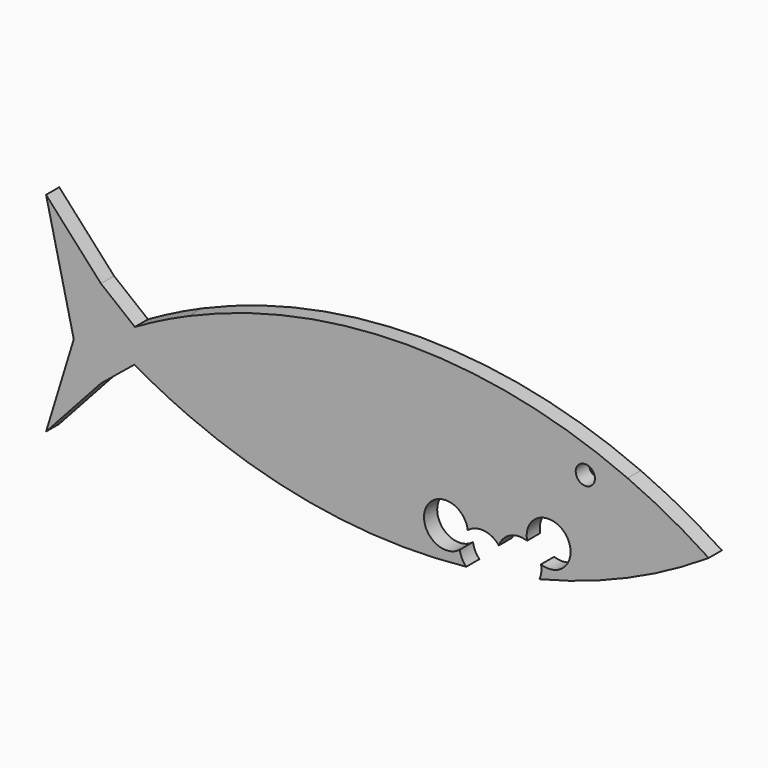
from build123d import *

# Parameters (mm, degrees)
F0_R     = 1.75
F1_DEPTH = 3


# Not quite as in the source:
# - a feature names something its author has since deleted; it is built from what else it names


with BuildPart() as f1:
    # F0 (on Front) → F1 (new body)
    with BuildSketch(Plane.XZ):
        with BuildLine():
            Line((0, 16), (0, 0))
            Line((0, 0), (43.6382221521, 0))
            ThreePointArc((43.6382221521, 0), (43.870370626, 0.294923121), (44.1291400161, 0.5667888304))
            ThreePointArc((44.1291400161, 0.5667888304), (41.7991534918, 8.3522131948), (44.5474305371, 16))
            Line((44.5474305371, 16), (0, 16))
        make_face()
        with BuildLine():
            ThreePointArc((-9.8901239272, 4.9856294086), (-5.0141391128, 2.3557845503), (0, 0))
            Line((0, 0), (0, 16))
            ThreePointArc((0, 16), (-4.9775998147, 13.6626256025), (-9.8191881817, 11.0551668638))
            ThreePointArc((-9.8191881817, 11.0551668638), (-12.3290859965, 9.5638999576), (-14.7943813031, 8))
            ThreePointArc((-14.7943813031, 8), (-12.3639476772, 6.4575177277), (-9.8901239272, 4.9856294086))
        make_face()
        with BuildLine():
            Line((43.6382221521, 0), (0, 0))
            ThreePointArc((0, 0), (24.7921839108, -7.1853331257), (50.5976363139, -7.7853510181))
            ThreePointArc((50.5976363139, -7.7853510181), (49.8103733831, -6.7032232406), (49.4240926583, -5.4219853039))
            ThreePointArc((49.4240926583, -5.4219853039), (44.1587611024, -5.2426073702), (43.6382221521, 0))
        make_face()
        with BuildLine():
            ThreePointArc((80, 16), (40, 24.3484861009), (0, 16))
            Line((0, 16), (44.5474305371, 16))
            ThreePointArc((44.5474305371, 16), (54.7943813031, 21), (65.041332069, 16))
            Line((65.041332069, 16), (80, 16))
        make_face()
        with BuildLine():
            Line((-16, -0.0001621457), (-9.8901239272, 4.9856294086))
            ThreePointArc((-9.8901239272, 4.9856294086), (-12.3639476772, 6.4575177277), (-14.7943813031, 8))
            ThreePointArc((-14.7943813031, 8), (-12.3290859965, 9.5638999576), (-9.8191881817, 11.0551668638))
            Line((-9.8191881817, 11.0551668638), (-16, 16))
            Line((-16, 16), (-16, -0.0001621457))
        make_face()
        with BuildLine():
            ThreePointArc((44.5474305371, 16), (41.7991534918, 8.3522131948), (44.1291400161, 0.5667888304))
            ThreePointArc((44.1291400161, 0.5667888304), (47.2688331903, 1.6585032514), (50.1496109619, 0))
            Line((50.1496109619, 0), (58.9824606658, 0))
            ThreePointArc((58.9824606658, 0), (60.2984076368, 0.2226618407), (61.6143546079, 0))
            Line((61.6143546079, 0), (61.6856141113, 0))
            ThreePointArc((61.6856141113, 0), (63.1331562403, 3.9268000172), (67.289866632, 4.41351894))
            ThreePointArc((67.289866632, 4.41351894), (67.6676347628, 6.1891037132), (67.7943813031, 8))
            ThreePointArc((67.7943813031, 8), (67.0868659981, 12.2302269468), (65.041332069, 16))
            Line((65.041332069, 16), (44.5474305371, 16))
        make_face()
        with BuildLine():
            ThreePointArc((65.041332069, 16), (54.7943813031, 21), (44.5474305371, 16))
            Line((44.5474305371, 16), (65.041332069, 16))
        make_face()
        with BuildLine():
            Line((80, 0), (80, 16))
            Line((80, 16), (65.041332069, 16))
            ThreePointArc((65.041332069, 16), (67.0868659981, 12.2302269468), (67.7943813031, 8))
            ThreePointArc((67.7943813031, 8), (67.6676347628, 6.1891037132), (67.289866632, 4.41351894))
            ThreePointArc((67.289866632, 4.41351894), (68.9789922296, 2.9374861341), (69.6079694957, 0.7843011149))
            ThreePointArc((69.6079694957, 0.7843011149), (69.5885110127, 0.3902335683), (69.53032488, 0))
            Line((69.53032488, 0), (80, 0))
        make_face()
        with Locations((72.2943813031, 14)):
            Circle(F0_R, mode=Mode.SUBTRACT)
        with BuildLine():
            ThreePointArc((94.7943813031, 8), (87.5656775591, 12.3115824444), (80, 16))
            Line((80, 16), (80, 0))
            ThreePointArc((80, 0), (87.5656775591, 3.6884175556), (94.7943813031, 8))
        make_face()
        Polygon((-26, -11.0001621457), (-16, -0.0001621457), (-16, 16), (-26, 27), (-20.9564695358, 5.4488921514), align=None)
        with BuildLine():
            Line((58.9824606658, 0), (50.1496109619, 0))
            ThreePointArc((50.1496109619, 0), (50.6198306879, -0.8687025049), (50.862827722, -1.8261486257))
            ThreePointArc((50.862827722, -1.8261486257), (53.8241968939, -0.9475550969), (56.5284231629, -2.4404697788))
            ThreePointArc((56.5284231629, -2.4404697788), (57.4778318355, -0.941081445), (58.9824606658, 0))
        make_face()
        with BuildLine():
            ThreePointArc((63.935726955, -5.4416422713), (72.0834406348, -3.0620164808), (80, 0))
            Line((80, 0), (69.53032488, 0))
            ThreePointArc((69.53032488, 0), (67.5568042663, -2.7088411721), (64.215128062, -2.965364569))
            ThreePointArc((64.215128062, -2.965364569), (64.2775332757, -3.3692215709), (64.2984076368, -3.7773381593))
            ThreePointArc((64.2984076368, -3.7773381593), (64.2066858557, -4.6290196511), (63.935726955, -5.4416422713))
        make_face()
    extrude(amount=F1_DEPTH)


solid = f1.part
